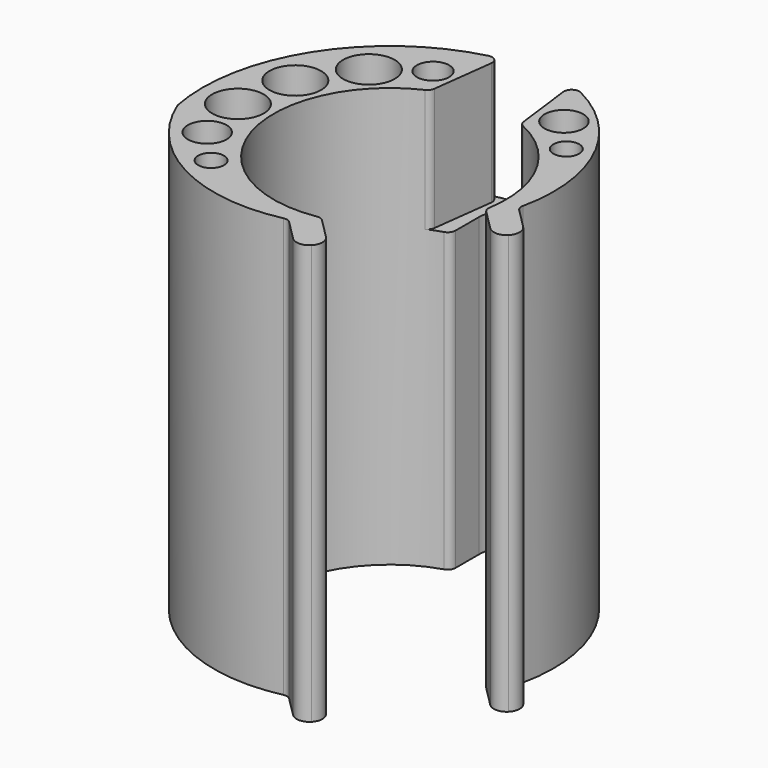
from build123d import *

# Parameters (mm, degrees)
F0_W     = 11
F0_H     = 65
F3_DEPTH = 19
F4_DEPTH = 65
F5_DEPTH = 65.001
F6_R     = 1.2
F7_R     = 1.99999
F2_R     = 2.5
F2_R_2   = 4
F2_R_3   = 3
F2_R_4   = 2
F8_DEPTH = 65.001


# Not quite as in the source:
# - a fillet or chamfer is up to 0.001 mm smaller than in the source, because OpenCascade refuses the exact size
# - a feature names something its author has since deleted; it is built from what else it names


with BuildPart() as f1:
    # F0 (on Front) → F1 (revolve)
    with BuildSketch(Plane.XZ):
        with Locations((-23.5, 0)):
            Rectangle(F0_W, F0_H)
    revolve(axis=Axis((0, 0, 0.8657751605), (0, 0, -1)))

    # F2 (on face) → F3 (cut)
    with BuildSketch(Plane.XY.offset(32.5)):
        with BuildLine():
            ThreePointArc((-4.5, 22.9), (0, 27.4), (4.5, 22.9))
            Line((4.5, 22.9), (4.5, 17.4284250579))
            ThreePointArc((4.5, 17.4284250579), (5.7655124222, 17.0516528967), (7, 16.5831239518))
            Line((7, 16.5831239518), (5.5, 28.4736720498))
            Line((5.5, 28.4736720498), (-5.5, 28.4736720498))
            Line((-5.5, 28.4736720498), (-7, 16.5831239518))
            ThreePointArc((-7, 16.5831239518), (-5.7655124222, 17.0516528967), (-4.5, 17.4284250579))
            Line((-4.5, 17.4284250579), (-4.5, 22.9))
        make_face()
        with BuildLine():
            Line((-5.5, 28.4736720498), (5.5, 28.4736720498))
            ThreePointArc((5.5, 28.4736720498), (0, 29), (-5.5, 28.4736720498))
        make_face()
        with BuildLine():
            ThreePointArc((17.6540730561, -3.5119374324), (12.7279220614, -12.7279220614), (3.5119374324, -17.6540730561))
            Line((3.5119374324, -17.6540730561), (8.4852813742, -22.627416998))
            Line((8.4852813742, -22.627416998), (5.6568542495, -25.4558441227))
            Line((5.6568542495, -25.4558441227), (2.1959599702, -28.916738402))
            ThreePointArc((2.1959599702, -28.916738402), (20.5060966544, -20.5060966544), (28.916738402, -2.1959599702))
            Line((28.916738402, -2.1959599702), (25.4558441227, -5.6568542495))
            Line((25.4558441227, -5.6568542495), (22.627416998, -8.4852813742))
            Line((22.627416998, -8.4852813742), (17.6540730561, -3.5119374324))
        make_face()
    extrude(amount=-F3_DEPTH, mode=Mode.SUBTRACT)

    # F2 (on face) → F4 (join, through all)
    with BuildSketch(Plane.XY.offset(32.5)):
        Polygon((8.4852813742, -22.627416998), (3.5119374324, -17.6540730561), (0.6835103076, -20.4825001809), (5.6568542495, -25.4558441227), align=None)
        with BuildLine():
            Line((5.6568542495, -25.4558441227), (0.6835103076, -20.4825001809))
            Line((0.6835103076, -20.4825001809), (-6.981162826, -28.1471733145))
            ThreePointArc((-6.981162826, -28.1471733145), (-2.4233446306, -28.8985709128), (2.1959599702, -28.916738402))
            Line((2.1959599702, -28.916738402), (5.6568542495, -25.4558441227))
        make_face()
        with BuildLine():
            ThreePointArc((2.1959599702, -28.916738402), (-2.4233446306, -28.8985709128), (-6.981162826, -28.1471733145))
            Line((-6.981162826, -28.1471733145), (-2.0078188841, -33.1205172564))
            Line((-2.0078188841, -33.1205172564), (2.1959599702, -28.916738402))
        make_face()
        Polygon((25.4558441227, -5.6568542495), (20.4825001809, -0.6835103076), (17.6540730561, -3.5119374324), (22.627416998, -8.4852813742), align=None)
        with BuildLine():
            Line((28.1471733145, 6.981162826), (20.4825001809, -0.6835103076))
            Line((20.4825001809, -0.6835103076), (25.4558441227, -5.6568542495))
            Line((25.4558441227, -5.6568542495), (28.916738402, -2.1959599702))
            ThreePointArc((28.916738402, -2.1959599702), (28.9791771248, -1.0987689344), (29, 0))
            ThreePointArc((29, 0), (28.7860037702, 3.5165305259), (28.1471733145, 6.981162826))
        make_face()
        with BuildLine():
            Line((33.1205172564, 2.0078188841), (28.1471733145, 6.981162826))
            ThreePointArc((28.1471733145, 6.981162826), (28.7860037702, 3.5165305259), (29, 0))
            ThreePointArc((29, 0), (28.9791771248, -1.0987689344), (28.916738402, -2.1959599702))
            Line((28.916738402, -2.1959599702), (33.1205172564, 2.0078188841))
        make_face()
    extrude(amount=-F4_DEPTH)

    # F2 (on face) → F5 (cut, through all)
    with BuildSketch(Plane.XY.offset(32.5)):
        with BuildLine():
            ThreePointArc((-4.5, 22.9), (0, 18.4), (4.5, 22.9))
            ThreePointArc((4.5, 22.9), (0, 27.4), (-4.5, 22.9))
        make_face()
        with BuildLine():
            Line((4.5, 17.4284250579), (4.5, 22.9))
            ThreePointArc((4.5, 22.9), (0, 18.4), (-4.5, 22.9))
            Line((-4.5, 22.9), (-4.5, 17.4284250579))
            ThreePointArc((-4.5, 17.4284250579), (0, 18), (4.5, 17.4284250579))
        make_face()
        with BuildLine():
            ThreePointArc((7, 16.5831239518), (5.7655124222, 17.0516528967), (4.5, 17.4284250579))
            ThreePointArc((4.5, 17.4284250579), (0, 18), (-4.5, 17.4284250579))
            ThreePointArc((-4.5, 17.4284250579), (-5.7655124222, 17.0516528967), (-7, 16.5831239518))
            Line((-7, 16.5831239518), (7, 16.5831239518))
        make_face()
        with BuildLine():
            ThreePointArc((28.1471733145, 6.981162826), (19.9628418868, 21.0353260921), (5.5, 28.4736720498))
            ThreePointArc((5.5, 28.4736720498), (18.4372066045, 16.6935009467), (20.4825001809, -0.6835103076))
            Line((20.4825001809, -0.6835103076), (28.1471733145, 6.981162826))
        make_face()
        with BuildLine():
            ThreePointArc((17.6540730561, -3.5119374324), (12.7279220614, -12.7279220614), (3.5119374324, -17.6540730561))
            Line((3.5119374324, -17.6540730561), (8.4852813742, -22.627416998))
            Line((8.4852813742, -22.627416998), (5.6568542495, -25.4558441227))
            Line((5.6568542495, -25.4558441227), (2.1959599702, -28.916738402))
            ThreePointArc((2.1959599702, -28.916738402), (20.5060966544, -20.5060966544), (28.916738402, -2.1959599702))
            Line((28.916738402, -2.1959599702), (25.4558441227, -5.6568542495))
            Line((25.4558441227, -5.6568542495), (22.627416998, -8.4852813742))
            Line((22.627416998, -8.4852813742), (17.6540730561, -3.5119374324))
        make_face()
        with BuildLine():
            Line((28.1471733145, 6.981162826), (20.4825001809, -0.6835103076))
            Line((20.4825001809, -0.6835103076), (25.4558441227, -5.6568542495))
            Line((25.4558441227, -5.6568542495), (28.916738402, -2.1959599702))
            ThreePointArc((28.916738402, -2.1959599702), (28.9791771248, -1.0987689344), (29, 0))
            ThreePointArc((29, 0), (28.7860037702, 3.5165305259), (28.1471733145, 6.981162826))
        make_face()
        with BuildLine():
            Line((33.1205172564, 2.0078188841), (28.1471733145, 6.981162826))
            ThreePointArc((28.1471733145, 6.981162826), (28.7860037702, 3.5165305259), (29, 0))
            ThreePointArc((29, 0), (28.9791771248, -1.0987689344), (28.916738402, -2.1959599702))
            Line((28.916738402, -2.1959599702), (33.1205172564, 2.0078188841))
        make_face()
        with BuildLine():
            Line((5.6568542495, -25.4558441227), (0.6835103076, -20.4825001809))
            Line((0.6835103076, -20.4825001809), (-6.981162826, -28.1471733145))
            ThreePointArc((-6.981162826, -28.1471733145), (-2.4233446306, -28.8985709128), (2.1959599702, -28.916738402))
            Line((2.1959599702, -28.916738402), (5.6568542495, -25.4558441227))
        make_face()
        with BuildLine():
            Line((-6.981162826, -28.1471733145), (0.6835103076, -20.4825001809))
            ThreePointArc((0.6835103076, -20.4825001809), (-16.6935009467, -18.4372066045), (-28.4736720498, -5.5))
            ThreePointArc((-28.4736720498, -5.5), (-21.0353260921, -19.9628418868), (-6.981162826, -28.1471733145))
        make_face()
        with BuildLine():
            ThreePointArc((2.1959599702, -28.916738402), (-2.4233446306, -28.8985709128), (-6.981162826, -28.1471733145))
            Line((-6.981162826, -28.1471733145), (-2.0078188841, -33.1205172564))
            Line((-2.0078188841, -33.1205172564), (2.1959599702, -28.916738402))
        make_face()
    extrude(amount=-F5_DEPTH, mode=Mode.SUBTRACT)

    # F6
    f6_edges = [f1.edges().sort_by_distance(p)[0] for p in [
        (3.511937, -17.654073, 0),
        (4.5, 17.428425, -9.5),
        (7, 16.583124, 23),
        (-7, 16.583124, 23),
        (-4.5, 17.428425, -9.5),
        (5.5, 28.473672, 23),
        (-5.5, 28.473672, 23),
        (0.68351, -20.4825, 0),
        (20.4825, -0.68351, 0),
        (17.654073, -3.511937, 0),
    ]]
    fillet(f6_edges, radius=F6_R)

    # F7 (radius 2 in the source; OpenCascade refuses exactly that, so slightly less here)
    f7_edges = [f1.edges().sort_by_distance(p)[0] for p in [
        (5.656854, -25.455844, 0),
        (8.485281, -22.627417, 0),
        (22.627417, -8.485281, 0),
        (25.455844, -5.656854, 0),
    ]]
    fillet(f7_edges, radius=F7_R)

    # F2 (on face) → F8 (cut, through all)
    with BuildSketch(Plane.XY.offset(32.5)):
        with Locations((-9.916601295, 20.7523738102)):
            Circle(F2_R)
        with Locations((-16.2634559673, 16.2634559673)):
            Circle(F2_R_2)
        with Locations((-21.397117557, 8.4358378511)):
            Circle(F2_R_2)
        with Locations((10.6623319362, 20.3792707839)):
            Circle(F2_R_3)
        with Locations((-22.9898786685, -0.6822600723)):
            Circle(F2_R_2)
        with Locations((-21.2449889591, -8.8119489404)):
            Circle(F2_R_3)
        with Locations((-16.2738828113, -14.2753784675)):
            Circle(F2_R_4)
        with Locations((15.4069372375, 14.9056833158)):
            Circle(F2_R_4)
    extrude(amount=-F8_DEPTH, mode=Mode.SUBTRACT)


solid = f1.part
